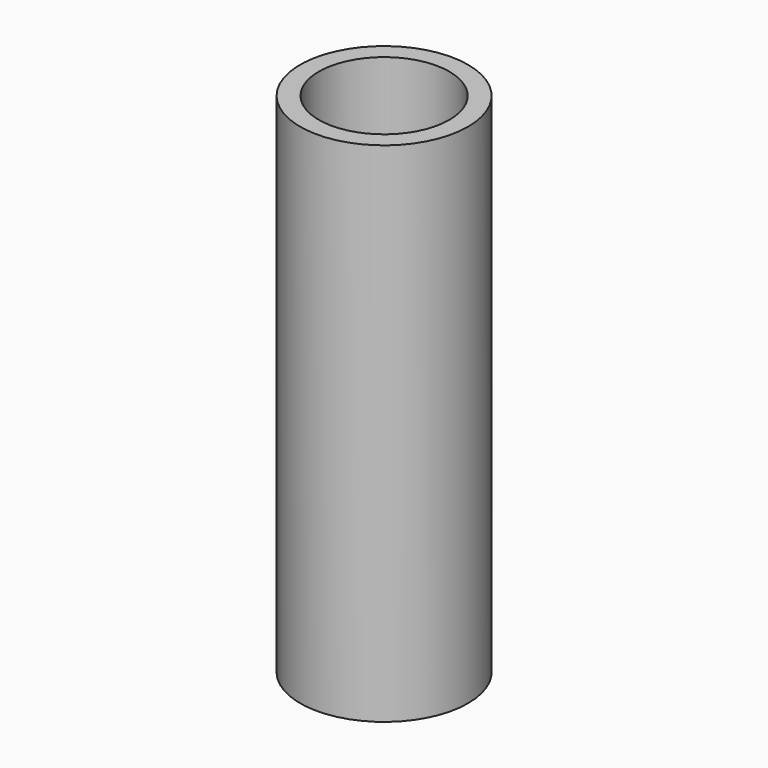
from build123d import *

# Parameters (mm, degrees)
F1_R     = 2.25
F1_R_2   = 1.75
F2_DEPTH = 13.6


with BuildPart() as f2:
    # F1 (on Top) → F2 (new body)
    with BuildSketch(Plane.XY):
        Circle(F1_R)
        Circle(F1_R_2, mode=Mode.SUBTRACT)
    extrude(amount=F2_DEPTH)


solid = f2.part
